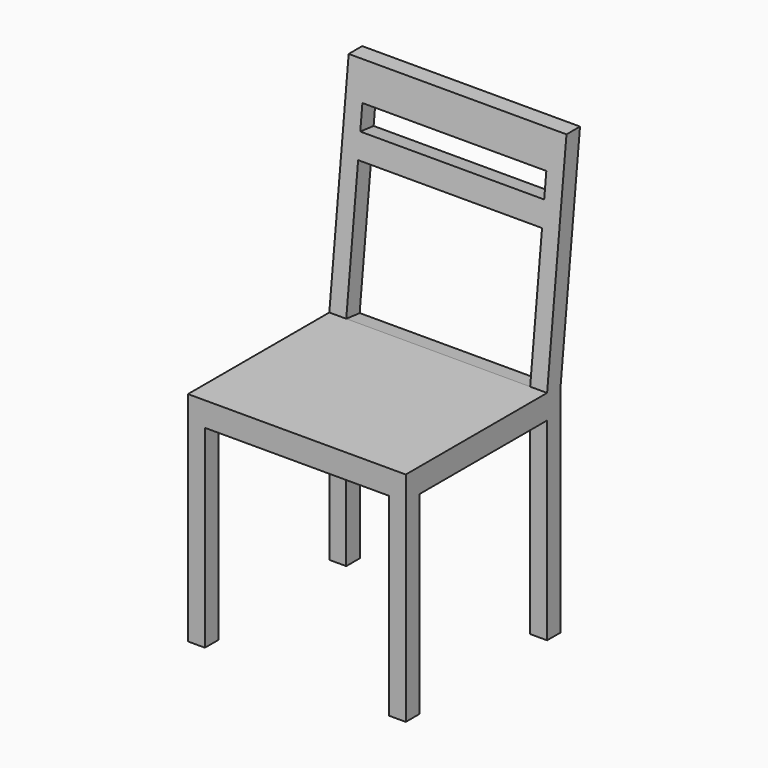
from build123d import *

# Parameters (mm, degrees)
F0_W     = 450
F0_H     = 900
F1_DEPTH = 225
F2_W     = 50
F2_H     = 50
F2_H_2   = 400
F2_W_2   = 330
F3_DEPTH = 450.001
F4_W     = 380
F4_H     = 400
F5_DEPTH = 450.001
F6_W     = 380
F6_H     = 277.7692569069
F6_H_2   = 50
F7_DEPTH = 134.1753041809


# Not quite as in the source:
# - a feature names something its author has since deleted; it is built from what else it names


with BuildPart() as f1:
    # F0 (on Front) → F1 (new body, symmetric)
    with BuildSketch(Plane.XZ):
        with Locations((0, 450)):
            Rectangle(F0_W, F0_H)
    extrude(amount=F1_DEPTH, both=True)

    # F2 (on face) → F3 (cut, through all)
    with BuildSketch(Plane.YZ.offset(225)):
        Polygon((-225, 450), (140, 450), (190, 900), (-225, 900), align=None)
        Polygon((175, 450), (225, 450), (225, 900), align=None)
        with Locations((200, 425)):
            Rectangle(F2_W, F2_H)
        with Locations((200, 200)):
            Rectangle(F2_W, F2_H_2)
        with Locations((-25, 200)):
            Rectangle(F2_W_2, F2_H_2)
    extrude(amount=-F3_DEPTH, mode=Mode.SUBTRACT)

    # F4 (on face) → F5 (cut, through all)
    with BuildSketch(Plane.XZ.offset(225)):
        with Locations((0, 200)):
            Rectangle(F4_W, F4_H)
    extrude(amount=-F5_DEPTH, mode=Mode.SUBTRACT)

    # F6 (on face) → F7 (cut, through all)
    with BuildSketch(Plane(origin=(0, 88.9024390244, -9.8780487805), x_dir=(1, 0, 0), z_dir=(0, -0.9938837347, 0.1104315261))):
        with Locations((0, 601.592722707)):
            Rectangle(F6_W, F6_H)
        with Locations((0, 815.4773511605)):
            Rectangle(F6_W, F6_H_2)
    extrude(amount=-F7_DEPTH, mode=Mode.SUBTRACT)


solid = f1.part
